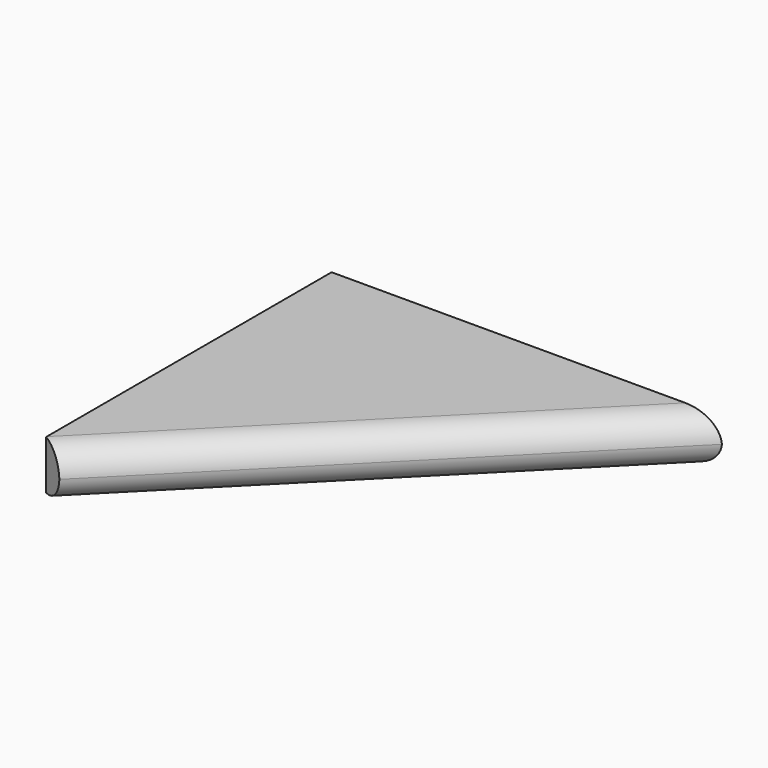
from build123d import *

# Parameters (mm, degrees)
F1_DEPTH    = 9.525
F2_T1_DEPTH = 126.6954628883


# Not quite as in the source:
# - a fillet or chamfer that OpenCascade refuses, or shapes differently, is made with other operations: its cross-section is extruded or revolved along the edge and cut away or added


with BuildPart() as f1:
    # F0 (on Top) → F1 (new body)
    with BuildSketch(Plane.XY):
        Polygon((0, 76.5490606427), (0, 7.1380194277), (4.5535564423, 4.6766349114), (75.9337022901, 76.5490606427), align=None)
    extrude(amount=F1_DEPTH)

    # F2: fillet of radius 5.08 on 2 edges, made by hand

    # F2_s2 → F2_t1 (cut)
    with BuildSketch(Plane(origin=(-4.3499505247, -4.3799503673, 0), x_dir=(0, 0, 1), z_dir=(0.7046726854, 0.7095325267, 0))):
        with BuildLine():
            ThreePointArc((5.08, -0.0646004733), (1.4878975516, -1.5524980249), (0, -5.1446004733))
            Line((0, -5.1446004733), (0, -0.0646004733))
            Line((0, -0.0646004733), (5.08, -0.0646004733))
        make_face()
        with BuildLine():
            ThreePointArc((4.445, -0.0646004733), (8.0371024484, -1.5524980249), (9.525, -5.1446004733))
            Line((9.525, -5.1446004733), (9.525, -0.0646004733))
            Line((9.525, -0.0646004733), (4.445, -0.0646004733))
        make_face()
    extrude(amount=F2_T1_DEPTH, mode=Mode.SUBTRACT)


solid = f1.part
